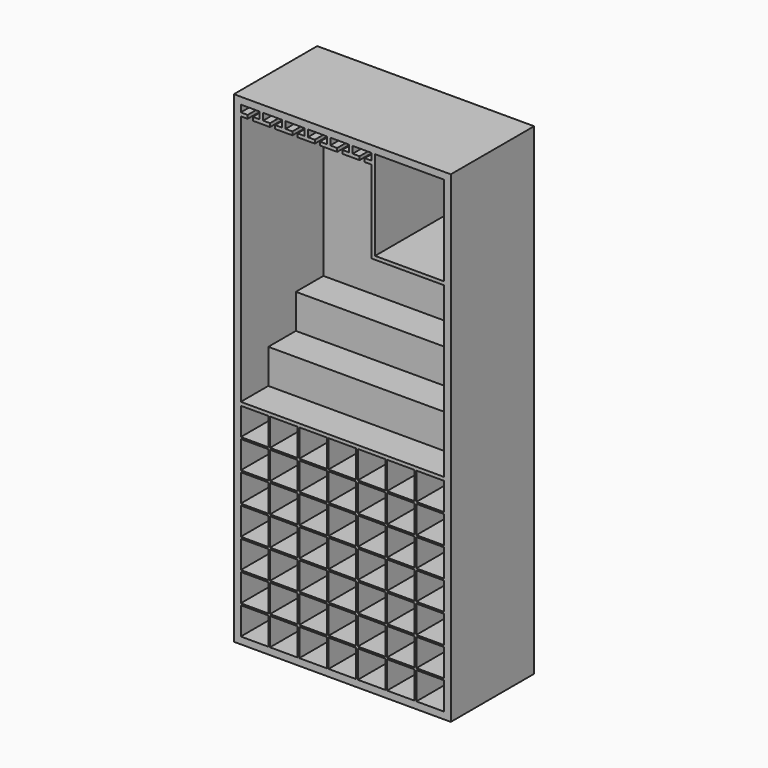
from build123d import *

# Parameters (mm, degrees)
F0_W      = 800.1
F0_H      = 1778
F0_W_2    = 749.3
F0_H_2    = 1727.2
F1_DEPTH  = 381
F2_W      = 800.1
F2_H      = 1778
F3_DEPTH  = 3.175
F4_W      = 101.6
F4_H      = 6.35
F5_DEPTH  = 381
F7_DEPTH  = 749.3
F8_W      = 25.4
F8_H      = 12.7
F9_DEPTH  = 381
F11_DEPTH = 381


with BuildPart() as f1:
    # F0 (on Front) → F1 (new body)
    with BuildSketch(Plane.XZ):
        with Locations((0, 889)):
            Rectangle(F0_W, F0_H)
        with Locations((0, 889)):
            Rectangle(F0_W_2, F0_H_2, mode=Mode.SUBTRACT)
    extrude(amount=-F1_DEPTH)

    # F2 (on face) → F3 (join)
    with BuildSketch(Plane(origin=(0, 381, 0), x_dir=(-1, 0, 0), z_dir=(0, 1, 0))):
        with Locations((0, 889)):
            Rectangle(F2_W, F2_H)
    extrude(amount=F3_DEPTH)

    # F4 (on face) → F5 (join, through all)
    with BuildSketch(Plane.XZ):
        with Locations((-323.85, 130.175)):
            Rectangle(F4_W, F4_H)
        with Locations((-323.85, 238.125)):
            Rectangle(F4_W, F4_H)
        with Locations((-323.85, 346.075)):
            Rectangle(F4_W, F4_H)
        with Locations((-323.85, 454.025)):
            Rectangle(F4_W, F4_H)
        with Locations((-323.85, 561.975)):
            Rectangle(F4_W, F4_H)
        with Locations((-323.85, 669.925)):
            Rectangle(F4_W, F4_H)
        with Locations((323.85, 669.925)):
            Rectangle(F4_W, F4_H)
        with Locations((323.85, 561.975)):
            Rectangle(F4_W, F4_H)
        with Locations((323.85, 454.025)):
            Rectangle(F4_W, F4_H)
        with Locations((323.85, 346.075)):
            Rectangle(F4_W, F4_H)
        with Locations((323.85, 238.125)):
            Rectangle(F4_W, F4_H)
        with Locations((323.85, 130.175)):
            Rectangle(F4_W, F4_H)
        Polygon((-266.7, 774.7), (-273.05, 774.7), (-273.05, 673.1), (-273.05, 666.75), (-273.05, 565.15), (-273.05, 558.8), (-273.05, 457.2), (-273.05, 450.85), (-273.05, 349.25), (-273.05, 342.9), (-273.05, 241.3), (-273.05, 234.95), (-273.05, 133.35), (-273.05, 127), (-273.05, 25.4), (-266.7, 25.4), (-266.7, 127), (-266.7, 133.35), (-266.7, 234.95), (-266.7, 241.3), (-266.7, 342.9), (-266.7, 349.25), (-266.7, 450.85), (-266.7, 457.2), (-266.7, 558.8), (-266.7, 565.15), (-266.7, 666.75), (-266.7, 673.1), align=None)
        Polygon((-158.75, 774.7), (-165.1, 774.7), (-165.1, 673.1), (-165.1, 666.75), (-165.1, 565.15), (-165.1, 558.8), (-165.1, 457.2), (-165.1, 450.85), (-165.1, 349.25), (-165.1, 342.9), (-165.1, 241.3), (-165.1, 234.95), (-165.1, 133.35), (-165.1, 127), (-165.1, 25.4), (-158.75, 25.4), (-158.75, 127), (-158.75, 133.35), (-158.75, 234.95), (-158.75, 241.3), (-158.75, 342.9), (-158.75, 349.25), (-158.75, 450.85), (-158.75, 457.2), (-158.75, 558.8), (-158.75, 565.15), (-158.75, 666.75), (-158.75, 673.1), align=None)
        Polygon((-50.8, 774.7), (-57.15, 774.7), (-57.15, 673.1), (-57.15, 666.75), (-57.15, 565.15), (-57.15, 558.8), (-57.15, 457.2), (-57.15, 450.85), (-57.15, 349.25), (-57.15, 342.9), (-57.15, 241.3), (-57.15, 234.95), (-57.15, 133.35), (-57.15, 127), (-57.15, 25.4), (-50.8, 25.4), (-50.8, 127), (-50.8, 133.35), (-50.8, 234.95), (-50.8, 241.3), (-50.8, 342.9), (-50.8, 349.25), (-50.8, 450.85), (-50.8, 457.2), (-50.8, 558.8), (-50.8, 565.15), (-50.8, 666.75), (-50.8, 673.1), align=None)
        Polygon((57.15, 774.7), (50.8, 774.7), (50.8, 673.1), (50.8, 666.75), (50.8, 565.15), (50.8, 558.8), (50.8, 457.2), (50.8, 450.85), (50.8, 349.25), (50.8, 342.9), (50.8, 241.3), (50.8, 234.95), (50.8, 133.35), (50.8, 127), (50.8, 25.4), (57.15, 25.4), (57.15, 127), (57.15, 133.35), (57.15, 234.95), (57.15, 241.3), (57.15, 342.9), (57.15, 349.25), (57.15, 450.85), (57.15, 457.2), (57.15, 558.8), (57.15, 565.15), (57.15, 666.75), (57.15, 673.1), align=None)
        Polygon((165.1, 673.1), (165.1, 774.7), (158.75, 774.7), (158.75, 673.1), (158.75, 666.75), (158.75, 565.15), (158.75, 558.8), (158.75, 457.2), (158.75, 450.85), (158.75, 349.25), (158.75, 342.9), (158.75, 241.3), (158.75, 234.95), (158.75, 133.35), (158.75, 127), (158.75, 25.4), (165.1, 25.4), (165.1, 127), (165.1, 133.35), (165.1, 234.95), (165.1, 241.3), (165.1, 342.9), (165.1, 349.25), (165.1, 450.85), (165.1, 457.2), (165.1, 558.8), (165.1, 565.15), (165.1, 666.75), align=None)
        Polygon((273.05, 673.1), (273.05, 774.7), (266.7, 774.7), (266.7, 673.1), (266.7, 666.75), (266.7, 565.15), (266.7, 558.8), (266.7, 457.2), (266.7, 450.85), (266.7, 349.25), (266.7, 342.9), (266.7, 241.3), (266.7, 234.95), (266.7, 133.35), (266.7, 127), (266.7, 25.4), (273.05, 25.4), (273.05, 127), (273.05, 133.35), (273.05, 234.95), (273.05, 241.3), (273.05, 342.9), (273.05, 349.25), (273.05, 450.85), (273.05, 457.2), (273.05, 558.8), (273.05, 565.15), (273.05, 666.75), align=None)
        with Locations((-215.9, 669.925)):
            Rectangle(F4_W, F4_H)
        with Locations((-107.95, 669.925)):
            Rectangle(F4_W, F4_H)
        with Locations((-215.9, 561.975)):
            Rectangle(F4_W, F4_H)
        with Locations((-215.9, 454.025)):
            Rectangle(F4_W, F4_H)
        with Locations((-107.95, 454.025)):
            Rectangle(F4_W, F4_H)
        with Locations((-107.95, 561.975)):
            Rectangle(F4_W, F4_H)
        with Locations((0, 561.975)):
            Rectangle(F4_W, F4_H)
        with Locations((0, 669.925)):
            Rectangle(F4_W, F4_H)
        with Locations((107.95, 669.925)):
            Rectangle(F4_W, F4_H)
        with Locations((107.95, 561.975)):
            Rectangle(F4_W, F4_H)
        with Locations((-215.9, 346.075)):
            Rectangle(F4_W, F4_H)
        with Locations((-215.9, 238.125)):
            Rectangle(F4_W, F4_H)
        with Locations((-215.9, 130.175)):
            Rectangle(F4_W, F4_H)
        with Locations((-107.95, 130.175)):
            Rectangle(F4_W, F4_H)
        with Locations((-107.95, 238.125)):
            Rectangle(F4_W, F4_H)
        with Locations((-107.95, 346.075)):
            Rectangle(F4_W, F4_H)
        with Locations((0, 346.075)):
            Rectangle(F4_W, F4_H)
        with Locations((107.95, 346.075)):
            Rectangle(F4_W, F4_H)
        with Locations((0, 238.125)):
            Rectangle(F4_W, F4_H)
        with Locations((0, 130.175)):
            Rectangle(F4_W, F4_H)
        with Locations((107.95, 130.175)):
            Rectangle(F4_W, F4_H)
        with Locations((215.9, 130.175)):
            Rectangle(F4_W, F4_H)
        with Locations((215.9, 238.125)):
            Rectangle(F4_W, F4_H)
        with Locations((107.95, 238.125)):
            Rectangle(F4_W, F4_H)
        with Locations((215.9, 346.075)):
            Rectangle(F4_W, F4_H)
        with Locations((215.9, 454.025)):
            Rectangle(F4_W, F4_H)
        with Locations((107.95, 454.025)):
            Rectangle(F4_W, F4_H)
        with Locations((0, 454.025)):
            Rectangle(F4_W, F4_H)
        with Locations((215.9, 561.975)):
            Rectangle(F4_W, F4_H)
        with Locations((215.9, 669.925)):
            Rectangle(F4_W, F4_H)
        Polygon((-374.65, 787.4), (-374.65, 774.7), (-273.05, 774.7), (-266.7, 774.7), (-165.1, 774.7), (-158.75, 774.7), (-57.15, 774.7), (-50.8, 774.7), (50.8, 774.7), (57.15, 774.7), (158.75, 774.7), (165.1, 774.7), (266.7, 774.7), (273.05, 774.7), (374.65, 774.7), (374.65, 787.4), align=None)
    extrude(amount=-F5_DEPTH)

    # F6 (on face) → F7 (join, through all)
    with BuildSketch(Plane.YZ.offset(-374.65)):
        Polygon((127, 914.4), (127, 787.4), (133.35, 787.4), (133.35, 908.05), (260.35, 908.05), (260.35, 1035.05), (381, 1035.05), (381, 1041.4), (254, 1041.4), (254, 914.4), align=None)
    extrude(amount=F7_DEPTH)

    # F8 (on face) → F9 (join, through all)
    with BuildSketch(Plane.XZ):
        Polygon((-292.1, 1752.6), (-304.8, 1752.6), (-304.8, 1727.2), (-330.2, 1727.2), (-330.2, 1714.5), (-266.7, 1714.5), (-266.7, 1727.2), (-292.1, 1727.2), align=None)
        Polygon((-247.65, 1727.2), (-247.65, 1714.5), (-184.15, 1714.5), (-184.15, 1727.2), (-209.55, 1727.2), (-209.55, 1752.6), (-222.25, 1752.6), (-222.25, 1727.2), align=None)
        Polygon((-165.1, 1727.2), (-165.1, 1714.5), (-101.6, 1714.5), (-101.6, 1727.2), (-127, 1727.2), (-127, 1752.6), (-139.7, 1752.6), (-139.7, 1727.2), align=None)
        Polygon((-82.55, 1727.2), (-82.55, 1714.5), (-19.05, 1714.5), (-19.05, 1727.2), (-44.45, 1727.2), (-44.45, 1752.6), (-57.15, 1752.6), (-57.15, 1727.2), align=None)
        Polygon((0, 1727.2), (0, 1714.5), (63.5, 1714.5), (63.5, 1727.2), (38.1, 1727.2), (38.1, 1752.6), (25.4, 1752.6), (25.4, 1727.2), align=None)
        with Locations((-361.95, 1720.85)):
            Rectangle(F8_W, F8_H)
    extrude(amount=-F9_DEPTH)

    # F10 (on face) → F11 (join, through all)
    with BuildSketch(Plane.XZ):
        Polygon((107.95, 1409.7), (374.65, 1409.7), (374.65, 1422.4), (120.65, 1422.4), (120.65, 1752.6), (107.95, 1752.6), (107.95, 1727.2), (82.55, 1727.2), (82.55, 1714.5), (107.95, 1714.5), align=None)
    extrude(amount=-F11_DEPTH)


solid = f1.part
